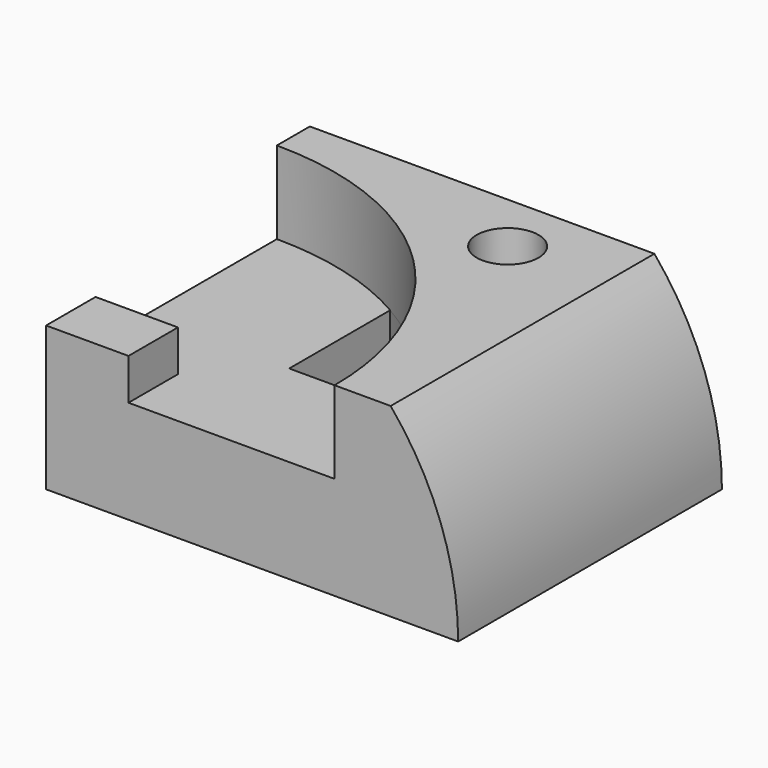
from build123d import *

# Parameters (mm, degrees)
F0_W      = 100
F0_H      = 80
F1_DEPTH  = 45
F3_DEPTH  = 20
F4_W      = 20
F4_H      = 15
F5_DEPTH  = 10
F7_DEPTH  = 25.001
F8_R      = 7.5
F9_DEPTH  = 30
F11_DEPTH = 80.001


# Not quite as in the source:
# - a feature names something its author has since deleted; it is built from what else it names


with BuildPart() as f1:
    # F0 (on Top) → F1 (new body)
    with BuildSketch(Plane.XY):
        with Locations((50, 40)):
            Rectangle(F0_W, F0_H)
    extrude(amount=F1_DEPTH)

    # F2 (on face) → F3 (cut)
    with BuildSketch(Plane.XY.offset(45)):
        with BuildLine():
            Line((0, 0), (70, 0))
            ThreePointArc((70, 0), (49.4974746831, 49.4974746831), (0, 70))
            Line((0, 70), (0, 0))
        make_face()
    extrude(amount=-F3_DEPTH, mode=Mode.SUBTRACT)

    # F4 (on face) → F5 (join)
    with BuildSketch(Plane.XY.offset(25)):
        with Locations((10, 7.5)):
            Rectangle(F4_W, F4_H)
    extrude(amount=F5_DEPTH)

    # F6 (on face) → F7 (cut, through all)
    with BuildSketch(Plane.XY.offset(25)):
        with BuildLine():
            Line((35, 60.6217782649), (35, 30))
            Line((35, 30), (63.2455532034, 30))
            ThreePointArc((63.2455532034, 30), (51.4535762322, 47.4608206094), (35, 60.6217782649))
        make_face()
    extrude(amount=-F7_DEPTH, mode=Mode.SUBTRACT)

    # F8 (on face) → F9 (cut)
    with BuildSketch(Plane.XY.offset(45)):
        with Locations((60, 65)):
            Circle(F8_R)
    extrude(amount=-F9_DEPTH, mode=Mode.SUBTRACT)

    # F10 (on face) → F11 (cut, through all)
    with BuildSketch(Plane.XZ):
        with BuildLine():
            ThreePointArc((83.6190264738, 45), (95.7773967757, 23.944395449), (100, 0))
            Line((100, 0), (100, 45))
            Line((100, 45), (83.6190264738, 45))
        make_face()
    extrude(amount=-F11_DEPTH, mode=Mode.SUBTRACT)


solid = f1.part
